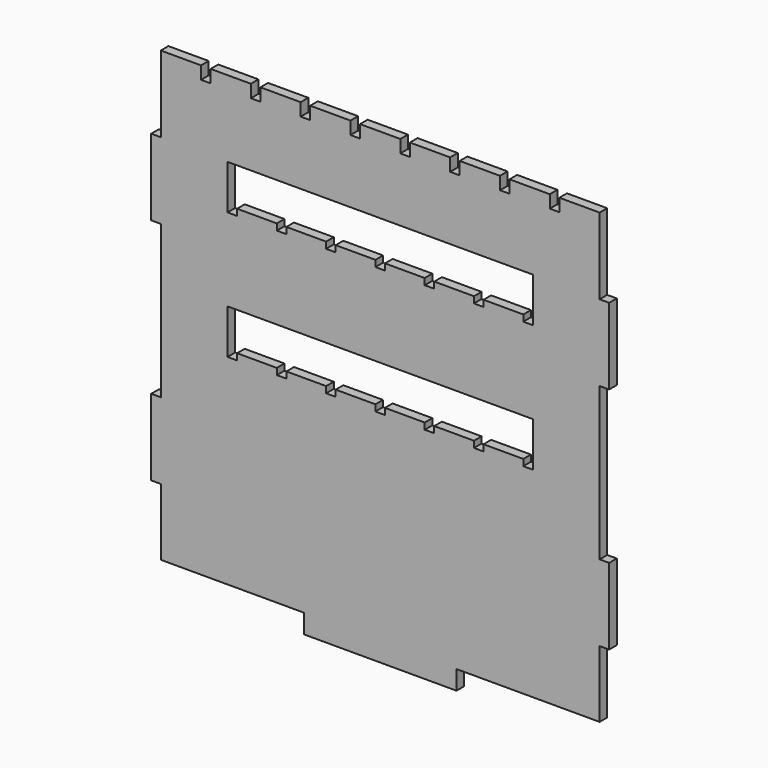
from build123d import *

# Parameters (mm, degrees)
F0_W     = 19.05
F0_H     = 152.4
F0_W_2   = 304.8
F0_H_2   = 38.1
F1_DEPTH = 19.05


# Not quite as in the source:
# - a feature names something its author has since deleted; it is built from what else it names


with BuildPart() as f1:
    # F0 (on Front) → F1 (new body)
    with BuildSketch(Plane.XZ):
        Polygon((-438.15, -314.325), (-438.15, -447.675), (-152.4, -447.675), (152.4, -447.675), (438.15, -447.675), (438.15, -314.325), (438.15, -161.925), (438.15, 142.875), (438.15, 295.275), (438.15, 447.675), (357.7166666667, 447.675), (357.7166666667, 422.275), (338.6666666667, 422.275), (338.6666666667, 447.675), (258.2333333333, 447.675), (258.2333333333, 422.275), (239.1833333333, 422.275), (239.1833333333, 447.675), (158.75, 447.675), (158.75, 422.275), (139.7, 422.275), (139.7, 447.675), (59.266836, 447.675), (59.266836, 422.275), (40.216836, 422.275), (40.216836, 447.675), (-40.216836, 447.675), (-40.216836, 422.275), (-59.266836, 422.275), (-59.266836, 447.675), (-139.7, 447.675), (-139.7, 422.275), (-158.75, 422.275), (-158.75, 447.675), (-239.1833333333, 447.675), (-239.1833333333, 422.275), (-258.2333333333, 422.275), (-258.2333333333, 447.675), (-338.6666666667, 447.675), (-338.6666666667, 422.275), (-357.7166666667, 422.275), (-357.7166666667, 447.675), (-438.15, 447.675), (-438.15, 295.275), (-438.15, 142.875), (-438.15, -161.925), align=None)
        Polygon((-304.8, -47.625), (-304.8, -34.925), (-304.8, 41.275), (304.8, 41.275), (304.8, -34.925), (304.8, -47.625), (285.75, -47.625), (285.75, -34.925), (206.375, -34.925), (206.375, -47.625), (187.325, -47.625), (187.325, -34.925), (107.95, -34.925), (107.95, -47.625), (88.9, -47.625), (88.9, -34.925), (9.525, -34.925), (9.525, -47.625), (-9.525, -47.625), (-9.525, -34.925), (-88.9, -34.925), (-88.9, -47.625), (-107.95, -47.625), (-107.95, -34.925), (-187.325, -34.925), (-187.325, -47.625), (-206.375, -47.625), (-206.375, -34.925), (-285.75, -34.925), (-285.75, -47.625), align=None, mode=Mode.SUBTRACT)
        Polygon((-304.8, 295.275), (304.8, 295.275), (304.8, 219.075), (304.8, 206.375), (285.75, 206.375), (285.75, 219.075), (206.375, 219.075), (206.375, 206.375), (187.325, 206.375), (187.325, 219.075), (107.95, 219.075), (107.95, 206.375), (88.9, 206.375), (88.9, 219.075), (9.525, 219.075), (9.525, 206.375), (-9.525, 206.375), (-9.525, 219.075), (-88.9, 219.075), (-88.9, 206.375), (-107.95, 206.375), (-107.95, 219.075), (-187.325, 219.075), (-187.325, 206.375), (-206.375, 206.375), (-206.375, 219.075), (-285.75, 219.075), (-285.75, 206.375), (-304.8, 206.375), (-304.8, 219.075), align=None, mode=Mode.SUBTRACT)
        with Locations((-447.675, 219.075)):
            Rectangle(F0_W, F0_H)
        with Locations((-447.675, -238.125)):
            Rectangle(F0_W, F0_H)
        with Locations((447.675, 219.075)):
            Rectangle(F0_W, F0_H)
        with Locations((447.675, -238.125)):
            Rectangle(F0_W, F0_H)
        with Locations((0, -466.725)):
            Rectangle(F0_W_2, F0_H_2)
    extrude(amount=F1_DEPTH)


solid = f1.part
